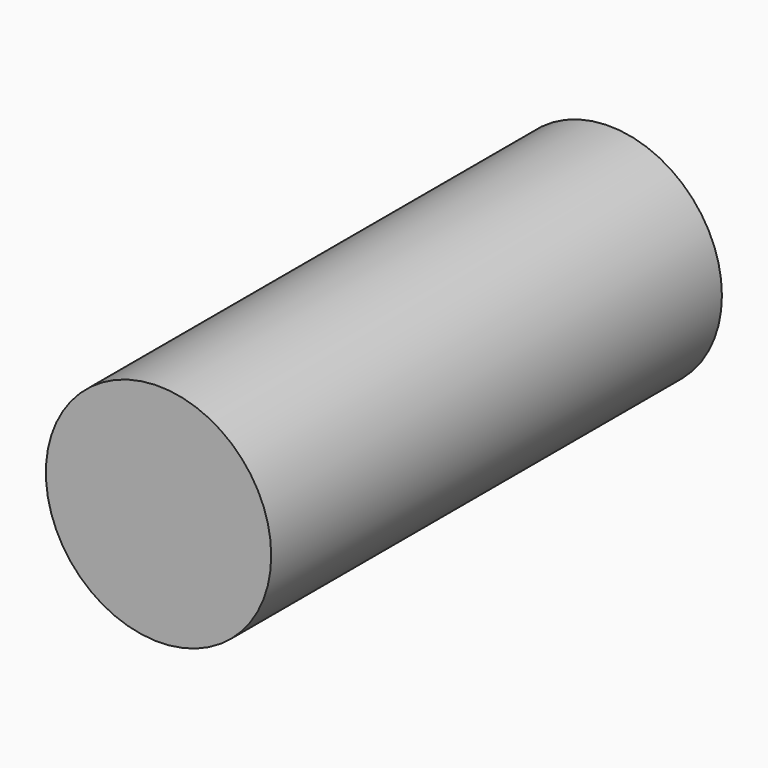
from build123d import *

# Parameters (mm, degrees)
F0_R     = 40
F1_DEPTH = 200
F2_R     = 40
F2_R_2   = 27.5
F3_DEPTH = 200


# Not quite as in the source:
# - a feature names something its author has since deleted; it is built from what else it names


with BuildPart() as f1:
    # F0 (on Front) → F1 (new body)
    with BuildSketch(Plane.XZ):
        Circle(F0_R)
    extrude(amount=F1_DEPTH)

    # F2 (on face) → F3 (join)
    with BuildSketch(Plane.XZ.offset(200)):
        Circle(F2_R)
        Circle(F2_R_2, mode=Mode.SUBTRACT)
        Circle(F2_R_2)
    extrude(amount=-F3_DEPTH)


solid = f1.part
